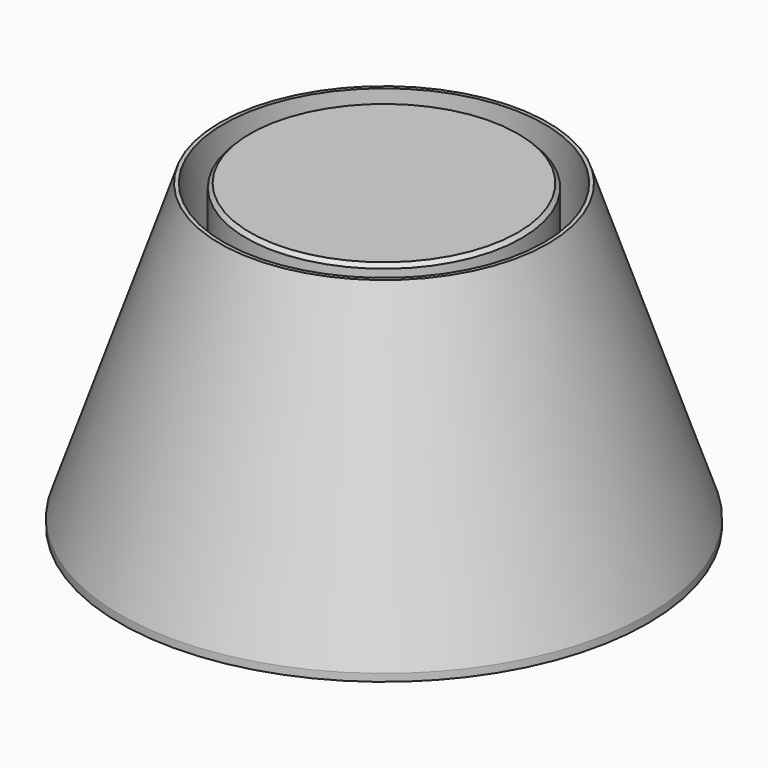
from build123d import *

# Parameters (mm, degrees)
F2_SIZE          = 1
F4_ANGLE_BACK    = 7.5
F4_ANGLE         = 15
F5_ANGLE_BACK    = 7.5
F5_ANGLE         = 15
F7_D             = 2.5
F7_DEPTH         = 15
F7_CSINK_D       = 5
F7_CSINK_ANGLE   = 45
F7_TIP           = 0.7510757738
F7_2_D           = 2.5
F7_2_DEPTH       = 15
F7_2_CSINK_D     = 5
F7_2_CSINK_ANGLE = 45
F7_2_TIP         = 0.7510757738
F8_R             = 5


with BuildPart() as f1:
    # F0 (on Front) → F1 (revolve)
    with BuildSketch(Plane.XZ):
        Polygon((70, 2), (43.5, 80), (42.5, 80), (42.5, 57), (36.5, 57), (36.5, 80), (31.5, 80), (0, 80), (0, 75), (31.5, 75), (31.5, 57), (31.5, 52.5413967947), (47.414124012, 52.5413967947), (59.3501898877, 18.2374222869), (63.9561501797, 5), (65, 2), (65, 0), (70, 0), align=None)
    revolve(axis=Axis((0, 0, 40), (0, 0, -1)))

    # F2
    f2_edges = [f1.edges().sort_by_distance(p)[0] for p in [
        (-36.5, 0, 80),
    ]]
    chamfer(f2_edges, length=F2_SIZE)

    # F0 (on Front) → F4 (revolve)
    with BuildSketch(Plane.XZ, mode=Mode.PRIVATE) as f4_sk:
        Polygon((51.8297031522, 5), (63.9561501797, 5), (59.3501898877, 18.2374222869), (51.8297031522, 18.2374222869), align=None)
    revolve(f4_sk.sketch.rotate(Axis((0, 0, 40), (0, 0, -1)), -F4_ANGLE_BACK), axis=Axis((0, 0, 40), (0, 0, -1)), revolution_arc=F4_ANGLE)

    # F0 (on Front) → F5 (revolve)
    with BuildSketch(Plane.XZ, mode=Mode.PRIVATE) as f5_sk:
        Polygon((-63.9561501797, 5), (-51.8297031522, 5), (-51.8297031522, 18.2374222869), (-59.3501898877, 18.2374222869), align=None)
    revolve(f5_sk.sketch.rotate(Axis((0, 0, 40), (0, 0, -1)), -F5_ANGLE_BACK), axis=Axis((0, 0, 40), (0, 0, -1)), revolution_arc=F5_ANGLE)

    # F7
    with Locations(Plane(origin=(0, 0, 0), x_dir=(1, 0, 0), z_dir=(0, 0, -1))):
        with Locations((58.2336969674, 0), (-58.4342479706, 0)):
            CounterSinkHole(F7_D / 2, F7_CSINK_D / 2, depth=F7_DEPTH, counter_sink_angle=F7_CSINK_ANGLE)
            with Locations((0, 0, -(F7_DEPTH + F7_TIP / 2))):  # 118° drill point
                Cone(0, F7_D / 2, F7_TIP, mode=Mode.SUBTRACT)

    # F8
    f8_edges = [f1.edges().sort_by_distance(p)[0] for p in [
        (-51.386293, -6.765134, 11.618711),
        (-51.386293, 6.765134, 11.618711),
        (51.386293, -6.765134, 11.618711),
        (51.386293, 6.765134, 11.618711),
        (-51.829703, 0, 18.237422),
        (51.829703, 0, 18.237422),
        (55.114367, 7.255944, 18.237422),
        (55.114367, -7.255944, 18.237422),
        (-55.114367, -7.255944, 18.237422),
        (-55.114367, 7.255944, 18.237422),
    ]]
    fillet(f8_edges, radius=F8_R)


with BuildPart() as f3:
    # F0 (on Front) → F3 (revolve)
    with BuildSketch(Plane.XZ):
        Polygon((0, 0), (65, 0), (65, 2), (63.9561501797, 5), (51.8297031522, 5), (0, 5), align=None)
    revolve(axis=Axis((0, 0, 40), (0, 0, -1)))

    # F7#2
    with Locations(Plane(origin=(0, 0, 0), x_dir=(1, 0, 0), z_dir=(0, 0, -1))):
        with Locations((58.2336969674, 0), (-58.4342479706, 0)):
            CounterSinkHole(F7_2_D / 2, F7_2_CSINK_D / 2, depth=F7_2_DEPTH, counter_sink_angle=F7_2_CSINK_ANGLE)
            with Locations((0, 0, -(F7_2_DEPTH + F7_2_TIP / 2))):  # 118° drill point
                Cone(0, F7_2_D / 2, F7_2_TIP, mode=Mode.SUBTRACT)


solid = Compound([f1.part, f3.part])
